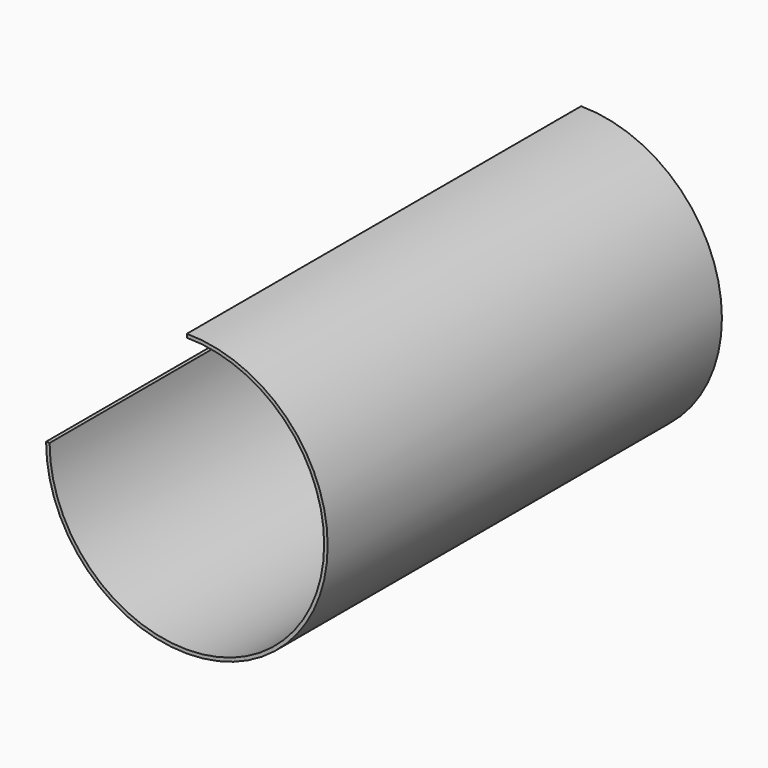
from build123d import *

# Parameters (mm, degrees)
F1_DEPTH = 350


# Not quite as in the source:
# - a feature of the source that left no trace in its solid (it failed there, or was rolled back) is left out
# - the program builds the solid bodies; features that only make, move or delete a surface that nothing else refers to are left out


with BuildPart() as f1:
    # F0 (on Front) → F1 (new body, symmetric)
    with BuildSketch(Plane.XZ):
        with BuildLine():
            Line((-195, 0), (-200, 0))
            ThreePointArc((-200, 0), (141.4213562373, -141.4213562373), (0, 200))
            Line((0, 200), (0, 195))
            ThreePointArc((0, 195), (137.8858223314, -137.8858223314), (-195, 0))
        make_face()
    extrude(amount=F1_DEPTH, both=True)


solid = f1.part
